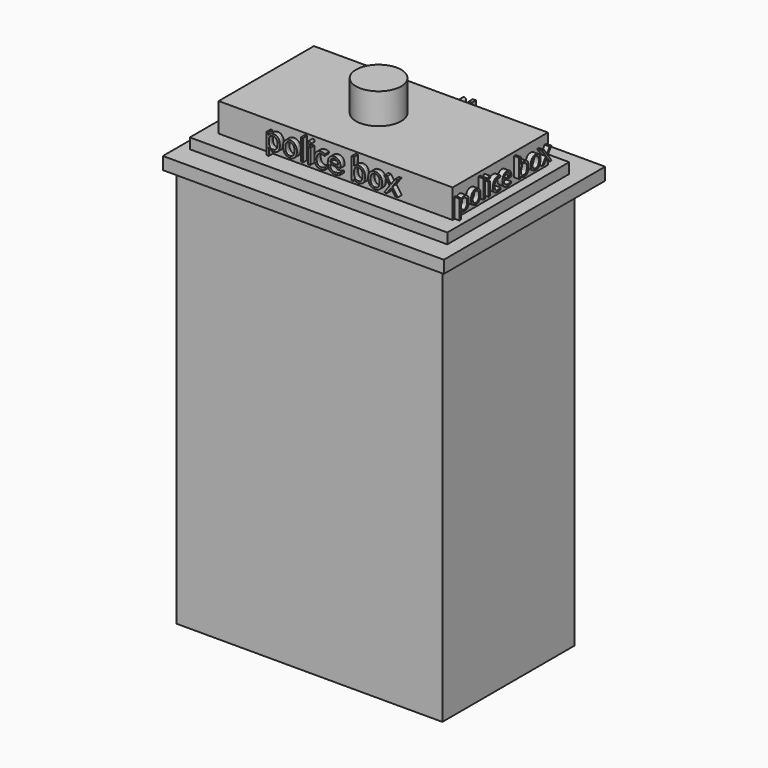
from build123d import *

# Parameters (mm, degrees)
F0_W          = 78.8445398211
F0_H          = 120.4411834478
F1_DEPTH      = 48.9
F3_W          = 83.2517407835
F3_H          = 59.7560126334
F4_DEPTH      = 3.7
F5_W          = 76.3022489846
F5_H          = 45.1523326337
F6_DEPTH      = 3.1
F7_W          = 69.3329479545
F7_H          = 35.2667816915
F8_DEPTH      = 8.5
F9_TEXT_SIZE  = 8.3579840769
F10_DEPTH     = 0.6
F11_R         = 6.6930703656
F12_DEPTH     = 9.1
F13_DEPTH     = 1.5
F14_TEXT_SIZE = 7.3388848261
F15_DEPTH     = 1.5
F16_TEXT_SIZE = 11.8055555556
F17_DEPTH     = 1.5


# Not quite as in the source:
# - Text() gives the source's letters only with a copy of the font that has no kerning and outlines rounded to 1/6400 em; it was checked with that copy


with BuildPart() as f1:
    # F0 (on Front) → F1 (new body)
    with BuildSketch(Plane.XZ):
        with Locations((6.4285695553, -2.7415975928)):
            Rectangle(F0_W, F0_H)
    extrude(amount=F1_DEPTH)

    # F3 (on offset) → F4 (join)
    with BuildSketch(Plane.XY.offset(55.9)):
        with Locations((6.8731997162, -21.7928839847)):
            Rectangle(F3_W, F3_H)
    extrude(amount=F4_DEPTH)

    # F5 (on face) → F6 (join)
    with BuildSketch(Plane.XY.offset(59.6)):
        with Locations((6.168121472, -22.5761663169)):
            Rectangle(F5_W, F5_H)
    extrude(amount=F6_DEPTH)

    # F7 (on face) → F8 (join)
    with BuildSketch(Plane.XY.offset(62.7)):
        with Locations((6.7203240469, -21.8689988833)):
            Rectangle(F7_W, F7_H)
    extrude(amount=F8_DEPTH)

    # F9 (on face) → F10 (join)
    with BuildSketch(Plane.XZ.offset(39.502389729)):
        with Locations((-13.2824879307, 64.3158557608)):
            Text('police box', F9_TEXT_SIZE, font='Open Sans', text_align=(TextAlign.LEFT, TextAlign.BOTTOM))
    extrude(amount=F10_DEPTH)

    # F11 (on face) → F12 (join)
    with BuildSketch(Plane.XY.offset(71.2)):
        with Locations((4.6515394934, -21.0188496858)):
            Circle(F11_R)
    extrude(amount=F12_DEPTH)

    # F9 (on face) → F13 (join)
    with BuildSketch(Plane.XZ.offset(39.502389729)):
        with Locations((-13.2824879307, 64.3158557608)):
            Text('police box', F9_TEXT_SIZE, font='Open Sans', text_align=(TextAlign.LEFT, TextAlign.BOTTOM))
    extrude(amount=F13_DEPTH)

    # F14 (on face) → F15 (join)
    with BuildSketch(Plane.YZ.offset(41.3867980242)):
        with Locations((-39.502389729, 64.5713995814)):
            Text('police box', F14_TEXT_SIZE, font='Open Sans', text_align=(TextAlign.LEFT, TextAlign.BOTTOM))
    extrude(amount=F15_DEPTH)

    # F16 (on face) → F17 (join)
    with BuildSketch(Plane(origin=(0, -4.2356080376, 0), x_dir=(-1, 0, 0), z_dir=(0, 1, 0))):
        with Locations((-34.2664324141, 62.7)):
            Text('police box', F16_TEXT_SIZE, font='Open Sans', text_align=(TextAlign.LEFT, TextAlign.BOTTOM))
    extrude(amount=F17_DEPTH)


solid = f1.part
